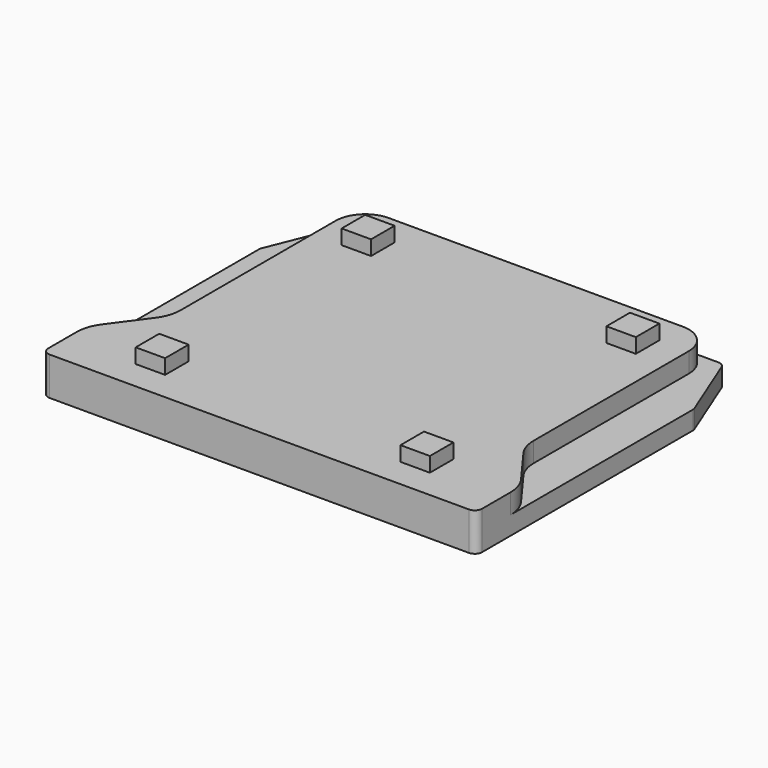
from build123d import *

# Parameters (mm, degrees)
F1_DEPTH    = 2.5
F3_DEPTH    = 2.7
F4_R        = 1
F5_R        = 5
F7_R        = 2
F8_DEPTH    = 1
F6_W        = 8
F6_H        = 15
F9_DEPTH    = 1.1
F10_SIZE2   = 1.09999
F10_SIZE    = 14.99999
F10_2_SIZE2 = 1.09999
F10_2_SIZE  = 14.99999
F13_W       = 4
F13_H       = 4
F14_DEPTH   = 2


# Not quite as in the source:
# - a fillet or chamfer that OpenCascade refuses, or shapes differently, is made with other operations: its cross-section is extruded or revolved along the edge and cut away or added
# - two fillets or chamfers of one size are made in one step
# - a fillet or chamfer is up to 0.001 mm smaller than in the source, because OpenCascade refuses the exact size


with BuildPart() as f1:
    # F0 (on Top) → F1 (new body)
    with BuildSketch(Plane.XY):
        Polygon((55, 0), (4, 0), (0, -10), (0, -47), (59, -47), (59, -10), align=None)
    extrude(amount=F1_DEPTH)

    # F2 (on face) → F3 (join)
    with BuildSketch(Plane.XY.offset(2.5)):
        with BuildLine():
            Line((0, -39.5), (0, -47))
            Line((0, -47), (59, -47))
            Line((59, -47), (59, -39.5))
            Line((59, -39.5), (53.5, -32))
            Line((53.5, -32), (53.5, -4))
            ThreePointArc((53.5, -4), (52.3284271247, -1.1715728753), (49.5, 0))
            Line((49.5, 0), (9.5, 0))
            ThreePointArc((9.5, 0), (6.6715728753, -1.1715728753), (5.5, -4))
            Line((5.5, -4), (5.5, -32))
            Line((5.5, -32), (0, -39.5))
        make_face()
    extrude(amount=F3_DEPTH)

    # F4
    f4_edges = [f1.edges().sort_by_distance(p)[0] for p in [
        (0, -47, 2.6),
        (59, -47, 2.6),
        (4, 0, 1.25),
        (55, 0, 1.25),
        (59, -10, 1.25),
        (0, -10, 1.25),
    ]]
    fillet(f4_edges, radius=F4_R)

    # F5
    f5_edges = [f1.edges().sort_by_distance(p)[0] for p in [
        (0, -39.5, 3.85),
        (59, -39.5, 3.85),
        (53.5, -32, 3.85),
        (5.5, -32, 3.85),
    ]]
    fillet(f5_edges, radius=F5_R)

    # F7 (on face) → F8 (cut)
    with BuildSketch(Plane(origin=(0, 0, 0), x_dir=(1, 0, 0), z_dir=(0, 0, -1))):
        with Locations((19, 20)):
            Circle(F7_R)
        with Locations((40, 20)):
            Circle(F7_R)
    extrude(amount=-F8_DEPTH, mode=Mode.SUBTRACT)

    # F6 (on face) → F9 (cut)
    with BuildSketch(Plane(origin=(0, 0, 0), x_dir=(1, 0, 0), z_dir=(0, 0, -1))):
        with Locations((40, 7.5)):
            Rectangle(F6_W, F6_H)
        with Locations((19, 7.5)):
            Rectangle(F6_W, F6_H)
    extrude(amount=-F9_DEPTH, mode=Mode.SUBTRACT)

    # F10 (size 15 and 1.1 in the source; OpenCascade refuses exactly that, so slightly less here)
    f10_edges = [f1.edges().sort_by_distance(p)[0] for p in [
        (40, -15, 1.1),
    ]]
    f10_side = f1.faces().sort_by_distance((40, -7.5, 1.1))[0]
    chamfer(f10_edges, length=F10_SIZE, length2=F10_SIZE2, reference=f10_side)

    # F10#2 (size 15 and 1.1 in the source; OpenCascade refuses exactly that, so slightly less here)
    f10_2_edges = [f1.edges().sort_by_distance(p)[0] for p in [
        (19, -15, 1.1),
    ]]
    f10_2_side = f1.faces().sort_by_distance((19, -7.5, 1.1))[0]
    chamfer(f10_2_edges, length=F10_2_SIZE, length2=F10_2_SIZE2, reference=f10_2_side)

    # F12: fillet of radius 2 on 2 edges, made by hand

    # F12_s1 → F12_t2 (revolve)
    with BuildSketch(Plane.XZ.offset(20)):
        with BuildLine():
            ThreePointArc((42, 0), (41.2679491924, 0.7320508076), (40.2679491924, 1))
            Line((40.2679491924, 1), (42, 1))
            Line((42, 1), (42, 0))
        make_face()
    revolve(axis=Axis((40, -20, 1), (0, 0, -1)))

    # F12_s3 → F12_t4 (revolve)
    with BuildSketch(Plane.XZ.offset(20)):
        with BuildLine():
            ThreePointArc((21, 0), (20.2679491924, 0.7320508076), (19.2679491924, 1))
            Line((19.2679491924, 1), (21, 1))
            Line((21, 1), (21, 0))
        make_face()
    revolve(axis=Axis((19, -20, 1), (0, 0, -1)))

    # F13 (on face) → F14 (join)
    with BuildSketch(Plane.XY.offset(5.2)):
        with Locations((11.5, -6)):
            Rectangle(F13_W, F13_H)
        with Locations((11.5, -41)):
            Rectangle(F13_W, F13_H)
        with Locations((47.5, -6)):
            Rectangle(F13_W, F13_H)
        with Locations((47.5, -41)):
            Rectangle(F13_W, F13_H)
    extrude(amount=F14_DEPTH)


solid = f1.part
